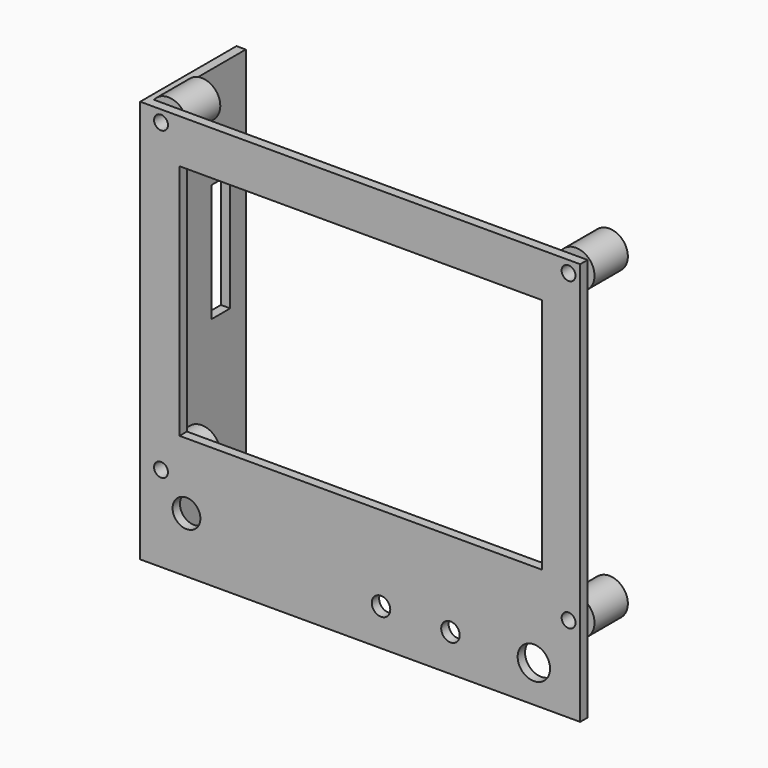
from build123d import *

# Parameters (mm, degrees)
F0_W     = 93
F0_H     = 87
F0_R     = 3
F0_R_2   = 2
F0_R_3   = 3.5
F0_W_2   = 78.25
F0_H_2   = 51.25
F1_DEPTH = 2
F2_R     = 4
F3_DEPTH = 9
F4_R     = 1.5
F5_DEPTH = 25
F6_W     = 26
F6_H     = 87
F6_W_2   = 5
F6_H_2   = 25.5
F7_DEPTH = 2


# Not quite as in the source:
# - a feature of the source that left no trace in its solid (it failed there, or was rolled back) is left out


with BuildPart() as f1:
    # F0 (on Front) → F1 (new body)
    with BuildSketch(Plane.XZ):
        Rectangle(F0_W, F0_H)
        with Locations((-38.5, -31.5)):
            Circle(F0_R, mode=Mode.SUBTRACT)
        with Locations((3.5, -35.5)):
            Circle(F0_R_2, mode=Mode.SUBTRACT)
        with Locations((18.5, -35.5)):
            Circle(F0_R_2, mode=Mode.SUBTRACT)
        with Locations((36.5, -35.5)):
            Circle(F0_R_3, mode=Mode.SUBTRACT)
        with Locations((-0.875, 8.375)):
            Rectangle(F0_W_2, F0_H_2, mode=Mode.SUBTRACT)
    extrude(amount=F1_DEPTH)

    # F2 (on face) → F3 (join)
    with BuildSketch(Plane(origin=(0, 0, 0), x_dir=(-1, 0, 0), z_dir=(0, 1, 0))):
        with Locations((-44, 41)):
            Circle(F2_R)
        with Locations((44, 41)):
            Circle(F2_R)
        with Locations((44, -25)):
            Circle(F2_R)
        with Locations((-44, -25)):
            Circle(F2_R)
    extrude(amount=F3_DEPTH)

    # F4 (on face) → F5 (cut)
    with BuildSketch(Plane(origin=(0, 9, 0), x_dir=(-1, 0, 0), z_dir=(0, 1, 0))):
        with Locations((-44, 41)):
            Circle(F4_R)
        with Locations((44, 41)):
            Circle(F4_R)
        with Locations((44, -25)):
            Circle(F4_R)
        with Locations((-44, -25)):
            Circle(F4_R)
    extrude(amount=-F5_DEPTH, mode=Mode.SUBTRACT)

    # F6 (on face) → F7 (join)
    with BuildSketch(Plane(origin=(-46.5, 0, 0), x_dir=(0, -1, 0), z_dir=(-1, 0, 0))):
        with Locations((-11, 0)):
            Rectangle(F6_W, F6_H)
        with Locations((-17.3, 8.75)):
            Rectangle(F6_W_2, F6_H_2, mode=Mode.SUBTRACT)
    extrude(amount=F7_DEPTH)


solid = f1.part
